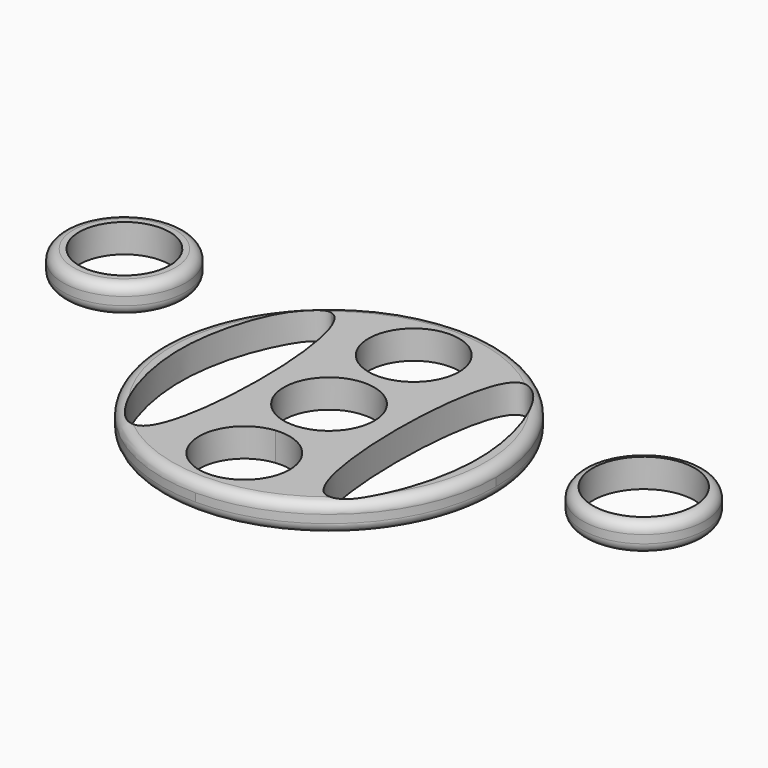
from build123d import *

# Parameters (mm, degrees)
F0_R      = 11.1
F1_DEPTH  = 7
F0_R_2    = 15
F0_R_3    = 12.5
F2_2_F1_R = 2.5
F2_2_F2_R = 2.5
F2_3_F1_R = 2.4999
F2_3_F2_R = 2.4999


# Not quite as in the source:
# - a fillet or chamfer that OpenCascade refuses, or shapes differently, is made with other operations: its cross-section is extruded or revolved along the edge and cut away or added
# - a fillet or chamfer is up to 0.001 mm smaller than in the source, because OpenCascade refuses the exact size
# - a feature names something its author has since deleted; it is built from what else it names


with BuildPart() as f1:
    # F0 (on Top) → F1 (new body)
    with BuildSketch(Plane.XY):
        with BuildLine():
            ThreePointArc((7.5, -12.9903810568), (12.9903810568, -7.5), (15, 0))
            ThreePointArc((15, 0), (12.9903810568, 7.5), (7.5, 12.9903810568))
            ThreePointArc((7.5, 12.9903810568), (4.4744589336, 14.3170952798), (1.2318753995, 14.9493305201))
            ThreePointArc((1.2318753995, 14.9493305201), (0, 14.8807621135), (-1.2318753995, 14.9493305201))
            ThreePointArc((-1.2318753995, 14.9493305201), (-4.4744589336, 14.3170952798), (-7.5, 12.9903810568))
            ThreePointArc((-7.5, 12.9903810568), (-15, 0), (-7.5, -12.9903810568))
            ThreePointArc((-7.5, -12.9903810568), (-4.4744589336, -14.3170952798), (-1.2318753995, -14.9493305201))
            ThreePointArc((-1.2318753995, -14.9493305201), (0, -14.8807621135), (1.2318753995, -14.9493305201))
            ThreePointArc((1.2318753995, -14.9493305201), (4.4744589336, -14.3170952798), (7.5, -12.9903810568))
        make_face()
        Circle(F0_R, mode=Mode.SUBTRACT)
        with BuildLine():
            ThreePointArc((7.5, 12.9903810568), (12.9903810568, 7.5), (15, 0))
            ThreePointArc((15, 0), (12.9903810568, -7.5), (7.5, -12.9903810568))
            ThreePointArc((7.5, -12.9903810568), (14.4888873943, -29.8630477901), (0, -40.9807621135))
            ThreePointArc((0, -40.9807621135), (28.9777747887, -28.9777747887), (40.9807621135, 0))
            ThreePointArc((40.9807621135, 0), (28.9777747809, 28.9777747965), (-2.21e-08, 40.9807621135))
            ThreePointArc((-2.21e-08, 40.9807621135), (14.4888873915, 29.8630478007), (7.5, 12.9903810568))
        make_face()
        with BuildLine():
            add(Edge.make_bspline(
                [(22, -29.1064200265), (14.9446387059, -22.6845711722), (14.9446387059, 22.6845711722), (22, 29.1064200265)],
                knots=[0.5991432693, 0.5991432693, 0.5991432693, 0.5991432693, 1, 1, 1, 1], degree=3))
            add(Edge.make_bspline(
                [(22, 29.1064200265), (27.2726721388, 33.9056503029), (45.6988520883, 0), (27.2726721388, -33.9056503029), (22, -29.1064200265)],
                knots=[0, 0, 0, 0, 0.2995716346, 0.5991432693, 0.5991432693, 0.5991432693, 0.5991432693], degree=3))
        make_face(mode=Mode.SUBTRACT)
        with BuildLine():
            ThreePointArc((1.2318753995, 14.9493305201), (4.4744589336, 14.3170952798), (7.5, 12.9903810568))
            ThreePointArc((7.5, 12.9903810568), (14.4888873915, 29.8630478007), (-2.21e-08, 40.9807621135))
            ThreePointArc((-2.21e-08, 40.9807621135), (-14.4888873972, 29.8630477794), (-7.5, 12.9903810568))
            ThreePointArc((-7.5, 12.9903810568), (-4.4744589336, 14.3170952798), (-1.2318753995, 14.9493305201))
            ThreePointArc((-1.2318753995, 14.9493305201), (-7.400546705, 34.25372461), (11.1, 25.9807621135))
            ThreePointArc((11.1, 25.9807621135), (8.2729624964, 18.5802154086), (1.2318753995, 14.9493305201))
        make_face()
        with BuildLine():
            ThreePointArc((0, -40.9807621135), (14.4888873943, -29.8630477901), (7.5, -12.9903810568))
            ThreePointArc((7.5, -12.9903810568), (4.4744589336, -14.3170952798), (1.2318753995, -14.9493305201))
            ThreePointArc((1.2318753995, -14.9493305201), (8.2729624964, -18.5802154086), (11.1, -25.9807621135))
            ThreePointArc((11.1, -25.9807621135), (-7.400546705, -34.25372461), (-1.2318753995, -14.9493305201))
            ThreePointArc((-1.2318753995, -14.9493305201), (-4.4744589336, -14.3170952798), (-7.5, -12.9903810568))
            ThreePointArc((-7.5, -12.9903810568), (-14.4888873943, -29.8630477901), (0, -40.9807621135))
        make_face()
        with BuildLine():
            ThreePointArc((-7.5, 12.9903810568), (-14.4888873972, 29.8630477794), (-2.21e-08, 40.9807621135))
            ThreePointArc((-2.21e-08, 40.9807621135), (-40.9807621135, -1.11e-08), (0, -40.9807621135))
            ThreePointArc((0, -40.9807621135), (-14.4888873943, -29.8630477901), (-7.5, -12.9903810568))
            ThreePointArc((-7.5, -12.9903810568), (-15, 0), (-7.5, 12.9903810568))
        make_face()
        with BuildLine():
            add(Edge.make_bspline(
                [(-22, 29.1064200265), (-27.2726721388, 33.9056503029), (-45.6988520883, 0), (-27.2726721388, -33.9056503029), (-22, -29.1064200265)],
                knots=[0, 0, 0, 0, 0.2995716346, 0.5991432693, 0.5991432693, 0.5991432693, 0.5991432693], degree=3))
            add(Edge.make_bspline(
                [(-22, -29.1064200265), (-14.9446387059, -22.6845711722), (-14.9446387059, 22.6845711722), (-22, 29.1064200265)],
                knots=[0.5991432693, 0.5991432693, 0.5991432693, 0.5991432693, 1, 1, 1, 1], degree=3))
        make_face(mode=Mode.SUBTRACT)
    extrude(amount=F1_DEPTH)

    # F2: fillet of radius 2.5 on 2 edges, made by hand

    # F2_s1 → F2_t2 (revolve, cut)
    with BuildSketch(Plane.YZ):
        with BuildLine():
            ThreePointArc((40.9807621135, 4.5), (40.2485290665, 6.267766953), (38.4807621135, 7))
            Line((38.4807621135, 7), (40.9807621135, 7))
            Line((40.9807621135, 7), (40.9807621135, 4.5))
        make_face()
    revolve(axis=Axis((0, 0, 7), (0, 0, 1)), mode=Mode.SUBTRACT)

    # F2_s3 → F2_t4 (revolve, cut)
    with BuildSketch(Plane.YZ):
        with BuildLine():
            ThreePointArc((40.9807621135, 2.5), (40.2485290665, 0.732233047), (38.4807621135, 0))
            Line((38.4807621135, 0), (40.9807621135, 0))
            Line((40.9807621135, 0), (40.9807621135, 2.5))
        make_face()
    revolve(axis=Axis((0, 0, 0), (0, 0, 1)), mode=Mode.SUBTRACT)


with BuildPart() as f1b:
    # F0 (on Top) → F1, piece 2 (new body)
    with BuildSketch(Plane.XY):
        with Locations((-70.8552226424, 25.8289314806)):
            Circle(F0_R_2)
        with Locations((-70.8552226424, 25.8289314806)):
            Circle(F0_R, mode=Mode.SUBTRACT)
    extrude(amount=F1_DEPTH)

    # F2#2: fillet of radius 2.5 on 2 edges, made by hand

    # F2_2_f1
    f2_2_f1_edges = [f1b.edges().sort_by_distance(p)[0] for p in [
        (-85.8552226424, 25.8289314806, 0),
    ]]
    fillet(f2_2_f1_edges, radius=F2_2_F1_R)

    # F2_2_f2
    f2_2_f2_edges = [f1b.edges().sort_by_distance(p)[0] for p in [
        (-85.8552226424, 25.8289314806, 7),
    ]]
    fillet(f2_2_f2_edges, radius=F2_2_F2_R)


with BuildPart() as f1c:
    # F0 (on Top) → F1, piece 3 (new body)
    with BuildSketch(Plane.XY):
        with Locations((68.5091763735, 10.8432136476)):
            Circle(F0_R_2)
        with Locations((68.5091763735, 10.8432136476)):
            Circle(F0_R_3, mode=Mode.SUBTRACT)
    extrude(amount=F1_DEPTH)

    # F2#3: fillet of radius 2.5 on 2 edges, made by hand

    # F2_3_f1 (radius 2.5 in the source; OpenCascade refuses exactly that, so slightly less here)
    f2_3_f1_edges = [f1c.edges().sort_by_distance(p)[0] for p in [
        (53.5091763735, 10.8432136476, 0),
    ]]
    fillet(f2_3_f1_edges, radius=F2_3_F1_R)

    # F2_3_f2 (radius 2.5 in the source; OpenCascade refuses exactly that, so slightly less here)
    f2_3_f2_edges = [f1c.edges().sort_by_distance(p)[0] for p in [
        (53.5091763735, 10.8432136476, 7),
    ]]
    fillet(f2_3_f2_edges, radius=F2_3_F2_R)


solid = Compound([f1.part, f1b.part, f1c.part])
